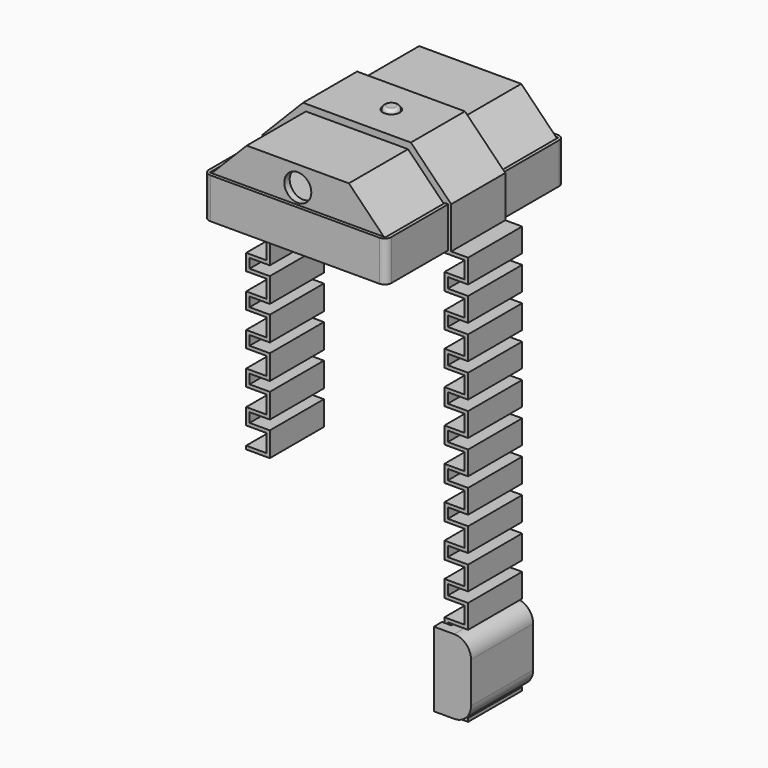
from build123d import *

# Parameters (mm, degrees)
F0_W      = 54
F0_H      = 66
F1_DEPTH  = 12
F2_T      = -2
F3_W      = 52
F3_H      = 64
F3_W_2    = 50
F3_H_2    = 62
F4_DEPTH  = 2
F5_W      = 51.8
F5_H      = 63.8
F6_DEPTH  = 1.5
F7_R      = 1.5
F7_W      = 3
F7_H      = 3
F8_DEPTH  = 2
F10_DEPTH = 5
F11_R     = 0.95
F12_DEPTH = 2
F14_DEPTH = 63.8
F15_T     = -2
F16_R     = 3.8140386686
F17_DEPTH = 1.5
F18_R     = 2
F19_W     = 1.1
F19_H     = 20
F20_DEPTH = 22.501
F22_DEPTH = 20
F23_R     = 4
F24_DEPTH = 2
F25_R     = 2.5
F26_DEPTH = 4.0009991715
F27_R     = 7
F27_R_2   = 5
F28_DEPTH = 2.5
F30_DEPTH = 20
F33_R     = 2.5
F34_DEPTH = 12.9999991715
F35_R     = 4.7500000565
F36_DEPTH = 3.5
F37_R     = 2.25
F38_DEPTH = 5
F39_R     = 1
F40_SIZE  = 2
F42_W     = 2
F42_H     = 1
F43_DEPTH = 20
F45_DEPTH = 20
F46_W     = 11
F46_H     = 22.0733063221
F47_DEPTH = 3
F48_W     = 3.5
F48_H     = 2
F49_DEPTH = 20
F50_R     = 5


# Not quite as in the source:
# - ends of sketch curves that miss each other by under 0.0002 mm in the source are joined


with BuildPart() as f1:
    # F0 (on Top) → F1 (new body)
    with BuildSketch(Plane.XY):
        Rectangle(F0_W, F0_H)
    extrude(amount=F1_DEPTH)

    # F2
    f2_openings = [f1.faces().sort_by_distance(p)[0] for p in [
        (0, 0, 12),
    ]]
    offset(amount=F2_T, openings=f2_openings)

    # F3 (on face) → F4 (cut)
    with BuildSketch(Plane.XY.offset(12)):
        Rectangle(F3_W, F3_H)
        Rectangle(F3_W_2, F3_H_2, mode=Mode.SUBTRACT)
    extrude(amount=-F4_DEPTH, mode=Mode.SUBTRACT)

    # F18
    f18_edges = [f1.edges().sort_by_distance(p)[0] for p in [
        (-27, 33, 6),
        (27, 33, 6),
        (27, -33, 6),
        (-27, -33, 6),
    ]]
    fillet(f18_edges, radius=F18_R)

    # F19 (on face) → F20 (cut, through all)
    with BuildSketch(Plane.XY):
        with Locations((26.45, 0)):
            Rectangle(F19_W, F19_H)
        with Locations((-26.45, 0)):
            Rectangle(F19_W, F19_H)
    extrude(amount=F20_DEPTH, mode=Mode.SUBTRACT)

    # F33 (on face) → F34 (cut, through all)
    with BuildSketch(Plane.XY.offset(24.4999991715)):
        with Locations((2.1, 0.1)):
            Circle(F33_R)
    extrude(amount=-F34_DEPTH, mode=Mode.SUBTRACT)


with BuildPart() as f6:
    # F5 (on face) → F6 (new body)
    with BuildSketch(Plane.XY.offset(10)):
        Rectangle(F5_W, F5_H)
    extrude(amount=F6_DEPTH)

    # F7 (on face) → F8 (join)
    with BuildSketch(Plane.XY.offset(11.5)):
        with Locations((-10.75, 27.25)):
            Circle(F7_R)
        with Locations((10.75, 27.25)):
            Circle(F7_R)
        with Locations((-11.35, -27.75)):
            Rectangle(F7_W, F7_H)
        with Locations((11.35, -27.75)):
            Rectangle(F7_W, F7_H)
    extrude(amount=F8_DEPTH)

    # F9 (on face) → F10 (join)
    with BuildSketch(Plane.XY.offset(11.5)):
        Polygon((-12.85, -29.25), (-12.85, -26.25), (-14.4459046423, -26.25), (-14.4459046423, -29.9), (-9.85, -29.9), (-9.85, -29.25), align=None)
        Polygon((12.85, -29.25), (9.85, -29.25), (9.85, -29.9), (14.4459046423, -29.9), (14.4459046423, -26.25), (12.85, -26.25), align=None)
    extrude(amount=F10_DEPTH)

    # F11 (on face) → F12 (join)
    with BuildSketch(Plane.XY.offset(13.5)):
        with Locations((-10.75, 27.25)):
            Circle(F11_R)
        with Locations((10.75, 27.25)):
            Circle(F11_R)
    extrude(amount=F12_DEPTH)

    # F16 (on face) → F17 (cut, through all)
    with BuildSketch(Plane.XY.offset(11.5)):
        with Locations((-16.7265478522, -20.9853146225)):
            Circle(F16_R)
    extrude(amount=-F17_DEPTH, mode=Mode.SUBTRACT)


with BuildPart() as f14:
    # F13 (on face) → F14 (new body, through all)
    with BuildSketch(Plane.XZ.offset(31.9)):
        Polygon((-25.9, 11.5), (25.9, 11.5), (15.1198767126, 22.5), (0, 22.5), (-15.1198767126, 22.5), align=None)
    extrude(amount=-F14_DEPTH)

    # F15
    f15_openings = [f14.faces().sort_by_distance(p)[0] for p in [
        (0, 0, 11.5),
    ]]
    offset(amount=F15_T, openings=f15_openings)

    # F23 (on face) → F24 (cut, through all)
    with BuildSketch(Plane.XZ.offset(31.9)):
        with Locations((0, 16.5)):
            Circle(F23_R)
    extrude(amount=-F24_DEPTH, mode=Mode.SUBTRACT)


with BuildPart() as f22:
    # F21 (on face) → F22 (new body, through all)
    with BuildSketch(Plane(origin=(0, -10, 0), x_dir=(-1, 0, 0), z_dir=(0, 1, 0))):
        Polygon((-25.9, 11.5), (-15.1198767126, 22.5), (15.1198767126, 22.5), (25.9, 11.5), (25.9, 10), (25.9, 0), (27.8999991715, 0), (27.8999991715, 10), (27.8999991715, 12.3166243929), (15.9601553379, 24.4999991715), (-15.9601553379, 24.4999991715), (-27.8999991715, 12.3166243929), (-27.8999991715, 10), (-27.8999991715, 0), (-25.9, 0), (-25.9, 10), align=None)
    extrude(amount=F22_DEPTH)


with BuildPart() as f26_tool:
    # F25 (on face) → F26 (new body, through all)
    with BuildSketch(Plane(origin=(0, 0, 20.5), x_dir=(1, 0, 0), z_dir=(0, 0, -1))):
        with Locations((2.1, -0.1)):
            Circle(F25_R)
    extrude(amount=-F26_DEPTH)


with BuildPart() as f14_1:
    add(f14.part)

    # F26: cut by f26_tool
    add(f26_tool.part, mode=Mode.SUBTRACT)

    # F27 (on face) → F28 (join)
    with BuildSketch(Plane(origin=(0, 0, 20.5), x_dir=(1, 0, 0), z_dir=(0, 0, -1))):
        with Locations((2.1, -0.1)):
            Circle(F27_R)
        with Locations((2.1, -0.1)):
            Circle(F27_R_2, mode=Mode.SUBTRACT)
    extrude(amount=F28_DEPTH)


with BuildPart() as f22_1:
    add(f22.part)

    # F26: cut by f26_tool
    add(f26_tool.part, mode=Mode.SUBTRACT)

    # F29 (on face) → F30 (join, through all)
    with BuildSketch(Plane.XZ.offset(10)):
        Polygon((27.9, 0), (25.9, 0), (25.9, -1), (31.9, -1), (31.9, -6), (25.9, -6), (25.9, -11), (31.9, -11), (31.9, -16), (25.9, -16), (25.9, -21), (31.9, -21), (31.9, -26), (25.9, -26), (25.9, -31), (31.9, -31), (31.9, -36), (25.9, -36), (25.9, -41), (31.9, -41), (31.9, -46), (25.9, -46), (25.9, -51), (31.9, -51), (31.9, -56), (25.9, -56), (25.9, -61), (31.9, -61), (31.9, -66), (25.9, -66), (25.9, -71), (31.9, -71), (31.9, -76), (25.9, -76), (25.9, -81), (31.9, -81), (32.9, -81), (32.9, -80), (26.9, -80), (26.9, -77), (32.9, -77), (32.9, -70), (26.9, -70), (26.9, -67), (32.9, -67), (32.9, -60), (26.9, -60), (26.9, -57), (32.9, -57), (32.9, -50), (26.9, -50), (26.9, -47), (32.9, -47), (32.9, -40), (26.9, -40), (26.9, -37), (32.9, -37), (32.9, -30), (26.9, -30), (26.9, -27), (32.9, -27), (32.9, -20), (26.9, -20), (26.9, -17), (32.9, -17), (32.9, -10), (26.9, -10), (26.9, -7), (32.9, -7), (32.9, 0), align=None)
        Polygon((32.9, -81), (31.9, -81), (31.9, -86), (25.9, -86), (25.9, -91), (31.9, -91), (31.9, -96), (25.9, -96), (25.9, -101), (31.9, -101), (31.9, -106), (25.9, -106), (25.9, -111), (31.9, -111), (31.9, -116), (25.9, -116), (25.9, -121), (31.9, -121), (32.9, -121), (32.9, -120), (26.9, -120), (26.9, -117), (32.9, -117), (32.9, -110), (26.9, -110), (26.9, -107), (32.9, -107), (32.9, -100), (26.9, -100), (26.9, -97), (32.9, -97), (32.9, -90), (26.9, -90), (26.9, -87), (32.9, -87), align=None)
        Polygon((-25.9, -1), (-25.9, 0), (-27.8999991715, 0), (-32.7999991715, 0), (-32.7999991715, -4.8), (-26.7999991715, -4.8), (-26.7999991715, -10.05), (-32.7999991715, -10.05), (-32.7999991715, -14.85), (-26.7999991715, -14.85), (-26.7999991715, -20.1), (-32.7999991715, -20.1), (-32.7999991715, -24.9), (-26.7999991715, -24.9), (-26.7999991715, -30.15), (-32.7999991715, -30.15), (-32.7999991715, -34.95), (-26.7999991715, -34.95), (-26.7999991715, -40.2), (-32.7999991715, -40.2), (-32.7999991715, -45), (-26.7999991715, -45), (-26.7999991715, -50.25), (-32.7999991715, -50.25), (-32.7999991715, -55.05), (-26.7999991715, -55.05), (-26.7999991715, -60.3), (-32.7999991715, -60.3), (-32.7999991715, -65.1), (-26.7999991715, -65.1), (-26.7999991715, -70.35), (-32.7999991715, -70.35), (-32.7999991715, -71.35), (-31.7999991715, -71.35), (-25.7999991715, -71.35), (-25.7999991715, -64.1), (-31.7999991715, -64.1), (-31.7999991715, -61.3), (-25.7999991715, -61.3), (-25.7999991715, -54.05), (-31.7999991715, -54.05), (-31.7999991715, -51.25), (-25.7999991715, -51.25), (-25.7999991715, -44), (-31.7999991715, -44), (-31.7999991715, -41.2), (-25.7999991715, -41.2), (-25.7999991715, -33.95), (-31.7999991715, -33.95), (-31.7999991715, -31.15), (-25.7999991715, -31.15), (-25.7999991715, -23.9), (-31.7999991715, -23.9), (-31.7999991715, -21.1), (-25.7999991715, -21.1), (-25.7999991715, -13.85), (-31.7999991715, -13.85), (-31.7999991715, -11.05), (-25.7999991715, -11.05), (-25.7999991715, -3.8), (-31.7999991715, -3.8), (-31.7999991715, -1), align=None)
    extrude(amount=-F30_DEPTH)

    # F42 (on face) → F43 (join, through all)
    with BuildSketch(Plane(origin=(0, 10, 0), x_dir=(-1, 0, 0), z_dir=(0, 1, 0))):
        with Locations((-24.9, -0.5)):
            Rectangle(F42_W, F42_H)
        with Locations((24.9, -0.5)):
            Rectangle(F42_W, F42_H)
    extrude(amount=-F43_DEPTH)


with BuildPart() as f36:
    # F35 (on face) → F36 (new body)
    with BuildSketch(Plane(origin=(0, 0, 20.5), x_dir=(1, 0, 0), z_dir=(0, 0, -1))):
        with Locations((2.1, -0.1)):
            Circle(F35_R)
    extrude(amount=F36_DEPTH)

    # F37 (on face) → F38 (join)
    with BuildSketch(Plane.XY.offset(20.5)):
        with Locations((2.1, 0.1)):
            Circle(F37_R)
    extrude(amount=F38_DEPTH)

    # F39
    f39_edges = [f36.edges().sort_by_distance(p)[0] for p in [
        (-0.15, 0.1, 25.5),
    ]]
    fillet(f39_edges, radius=F39_R)

    # F40
    f40_edges = [f36.edges().sort_by_distance(p)[0] for p in [
        (-2.65, 0.1, 17),
    ]]
    chamfer(f40_edges, length=F40_SIZE)


with BuildPart() as f45:
    # F44 (on face) → F45 (new body, through all)
    with BuildSketch(Plane.XZ.offset(10)):
        Polygon((36.1636182964, -97.463346839), (27.9010012746, -97.463346839), (27.9010012746, -99.4877822797), (33.1636182964, -99.4877822797), (33.1636182964, -107.4877822797), (27.9010012746, -107.4877822797), (27.9010012746, -109.5122177203), (33.1636182964, -109.5122177203), (33.1636182964, -117.5122177203), (27.9010012746, -117.5122177203), (27.9010012746, -119.536653161), (36.1636182964, -119.536653161), align=None)
    extrude(amount=-F45_DEPTH)

    # F46 (on face) → F47 (join)
    with BuildSketch(Plane.XZ.offset(10)):
        with Locations((30.6636182964, -108.5)):
            Rectangle(F46_W, F46_H)
    extrude(amount=F47_DEPTH)

    # F48 (on face) → F49 (join, through all)
    with BuildSketch(Plane(origin=(0, -10, 0), x_dir=(-1, 0, 0), z_dir=(0, 1, 0))):
        with Locations((-26.9136182964, -113.5122177203)):
            Rectangle(F48_W, F48_H)
        with Locations((-26.9136182964, -103.4877822797)):
            Rectangle(F48_W, F48_H)
    extrude(amount=F49_DEPTH)

    # F50
    f50_edges = [f45.edges().sort_by_distance(p)[0] for p in [
        (36.163618, -1.5, -97.463347),
        (36.163618, -1.5, -119.536653),
    ]]
    fillet(f50_edges, radius=F50_R)


solid = Compound([f1.part, f6.part, f14_1.part, f22_1.part, f36.part, f45.part])
